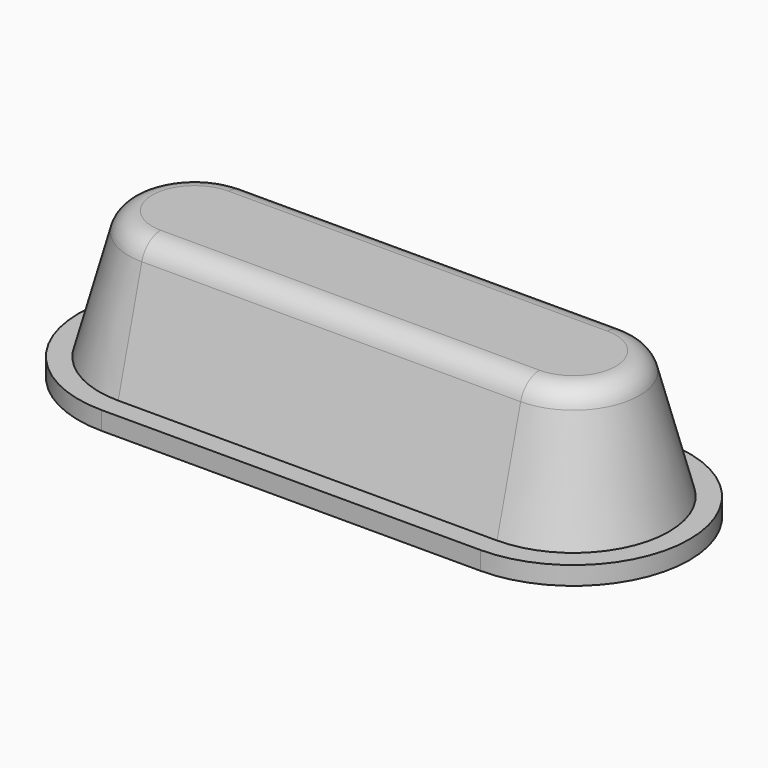
from build123d import *

# Parameters (mm, degrees)
F1_DEPTH     = 1.5
F3_DEPTH     = 10.5
F4_T4_DEPTH  = 31
F4_T9_ANGLE  = 180
F4_T14_DEPTH = 31
F4_T19_ANGLE = 180
F5_T         = 2.5
F5_T3_DEPTH  = 36
F5_T6_ANGLE  = 180.000000001
F5_T8_ANGLE  = 180.000000001
F6_R         = 2


# Not quite as in the source:
# - a fillet or chamfer that OpenCascade refuses, or shapes differently, is made with other operations: its cross-section is extruded or revolved along the edge and cut away or added
# - a shell that OpenCascade refuses in one call is made with other operations: the cavity is built on its own and cut out


with BuildPart() as f1:
    # F0 (on Top) → F1 (new body)
    with BuildSketch(Plane.XY):
        with BuildLine():
            Line((15.5, 9.5), (-15.5, 9.5))
            ThreePointArc((-15.5, 9.5), (-25, 0), (-15.5, -9.5))
            Line((-15.5, -9.5), (15.5, -9.5))
            ThreePointArc((15.5, -9.5), (25, 0), (15.5, 9.5))
        make_face()
        with BuildLine():
            ThreePointArc((-15.5, -8), (-23.5, 0), (-15.5, 8))
            Line((-15.5, 8), (15.5, 8))
            ThreePointArc((15.5, 8), (23.5, 0), (15.5, -8))
            Line((15.5, -8), (-15.5, -8))
        make_face(mode=Mode.SUBTRACT)
        with BuildLine():
            Line((15.5, 8), (-15.5, 8))
            ThreePointArc((-15.5, 8), (-23.5, 0), (-15.5, -8))
            Line((-15.5, -8), (15.5, -8))
            ThreePointArc((15.5, -8), (23.5, 0), (15.5, 8))
        make_face()
    extrude(amount=-F1_DEPTH)

    # F2 (on face) → F3 (join)
    with BuildSketch(Plane.XY):
        with BuildLine():
            Line((15.5, 8), (-15.5, 8))
            ThreePointArc((-15.5, 8), (-23.5, 0), (-15.5, -8))
            Line((-15.5, -8), (15.5, -8))
            ThreePointArc((15.5, -8), (23.5, 0), (15.5, 8))
        make_face()
    extrude(amount=F3_DEPTH)

    # F4: chamfer of 3 x 11.1961524227 on 4 edges, made by hand


with BuildPart() as f4_tool2:
    # F4_s3 → F4_t4 (new body)
    with BuildSketch(Plane.YZ.offset(-15.5)):
        Polygon((-8, -0.6961524227), (-5, 10.5), (-8, 10.5), align=None)
    extrude(amount=F4_T4_DEPTH)

    split(bisect_by=Plane.XY, keep=Keep.TOP)


with BuildPart() as f1_1:
    add(f1.part)

    # F4_t1: cut F4_tool2
    add(f4_tool2.part, mode=Mode.SUBTRACT)


with BuildPart() as f4_tool7:
    # F4_s8 → F4_t9 (revolve)
    with BuildSketch(Plane.YZ.offset(15.5)):
        Polygon((-8, -0.6961524227), (-5, 10.5), (-8, 10.5), align=None)
    revolve(axis=Axis((15.5, 0, 10.5), (0, 0, 1)), revolution_arc=F4_T9_ANGLE)

    split(bisect_by=Plane.XY, keep=Keep.TOP)


with BuildPart() as f1_2:
    add(f1_1.part)

    # F4_t6: cut F4_tool7
    add(f4_tool7.part, mode=Mode.SUBTRACT)


with BuildPart() as f4_tool12:
    # F4_s13 → F4_t14 (new body)
    with BuildSketch(Plane.YZ.offset(15.5)):
        Polygon((8, -0.6961524227), (5, 10.5), (8, 10.5), align=None)
    extrude(amount=-F4_T14_DEPTH)

    split(bisect_by=Plane.XY, keep=Keep.TOP)


with BuildPart() as f1_3:
    add(f1_2.part)

    # F4_t11: cut F4_tool12
    add(f4_tool12.part, mode=Mode.SUBTRACT)


with BuildPart() as f4_tool17:
    # F4_s18 → F4_t19 (revolve)
    with BuildSketch(Plane.YZ.offset(-15.5)):
        Polygon((8, -0.6961524227), (5, 10.5), (8, 10.5), align=None)
    revolve(axis=Axis((-15.5, 0, 10.5), (0, 0, 1)), revolution_arc=F4_T19_ANGLE)

    split(bisect_by=Plane.XY, keep=Keep.TOP)


with BuildPart() as f1_4:
    add(f1_3.part)

    # F4_t16: cut F4_tool17
    add(f4_tool17.part, mode=Mode.SUBTRACT)

    # F5: shell of thickness 2.5, made by hand


with BuildPart() as f5_core1:
    # F5_t2: copy of F1
    add(f1_4.part)

    # the walls: a layer under each face that stays
    f5_faces = [f5_core1.faces().sort_by_distance(p)[0] for p in [
        (25, 0, -0.75),
        (0, -9.5, -0.75),
        (0, 9.5, -0.75),
        (-21.4285714286, -5.4285714286, 0),
        (-25, 0, -0.75),
        (0, -6.4067332603, 5.25),
        (0, 6.4067332603, 5.25),
        (21.9067332603, 0, 5.25),
        (-21.9067332603, 0, 5.25),
        (0, 0, 10.5),
    ]]
    thicken(f5_faces, amount=-F5_T, mode=Mode.SUBTRACT)

    # F5_s4 → F5_t3 (cut)
    with BuildSketch(Plane.YZ.offset(-18)):
        Polygon((-7.8376146662, 0.0314704761), (-7.8134665205, -2.5), (-5.8951490506, -2.5), (-5.3986519548, -0.6470476128), align=None)
        Polygon((7.8376146662, 0.0314704761), (7.8134665205, -2.5), (5.8951490506, -2.5), (5.3986519548, -0.6470476128), align=None)
    extrude(amount=F5_T3_DEPTH, mode=Mode.SUBTRACT)

    # F5_s5 → F5_t6 (revolve, cut)
    with BuildSketch(Plane.YZ.offset(-15.5)):
        Polygon((7.8376146662, 0.0314704761), (7.8134665205, -2.5), (5.8951490506, -2.5), (5.3986519548, -0.6470476128), align=None)
    revolve(axis=Axis((-15.5, 0, 0), (0, 0, 1)), revolution_arc=F5_T6_ANGLE, mode=Mode.SUBTRACT)

    # F5_s7 → F5_t8 (revolve, cut)
    with BuildSketch(Plane.YZ.offset(15.5)):
        Polygon((-7.8376146662, 0.0314704761), (-7.8134665205, -2.5), (-5.8951490506, -2.5), (-5.3986519548, -0.6470476128), align=None)
    revolve(axis=Axis((15.5, 0, 0), (0, 0, 1)), revolution_arc=F5_T8_ANGLE, mode=Mode.SUBTRACT)


with BuildPart() as f1_5:
    add(f1_4.part)

    # what is left inside the walls is the cavity
    f5_cavity = [f5_core1.part.solids().sort_by_distance(p)[0] for p in [
        (0, -1.875733, -1.475),
    ]]
    add(f5_cavity, mode=Mode.SUBTRACT)

    # F6
    f6_edges = [f1_5.edges().sort_by_distance(p)[0] for p in [
        (-20.5, 0, 10.5),
    ]]
    fillet(f6_edges, radius=F6_R)


solid = f1_5.part
